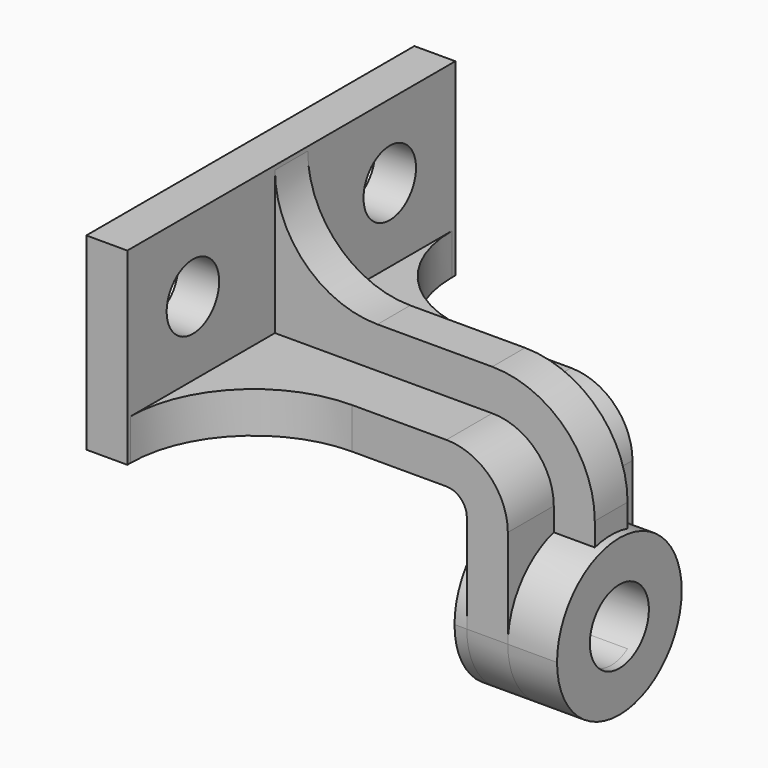
from build123d import *

# Parameters (mm, degrees)
F0_W      = 10
F0_H      = 36
F0_H_2    = 10
F0_W_2    = 58
F0_H_3    = 48
F1_DEPTH  = 50
F4_DEPTH  = 58.001
F2_R      = 8
F5_DEPTH  = 25
F6_R      = 15
F7_R      = 5
F9_DEPTH  = 5
F10_R     = 25
F13_DEPTH = 25
F12_R     = 9
F14_DEPTH = 25
F15_DEPTH = 25


# Not quite as in the source:
# - after a boolean that leaves OpenCascade's solid faulty, fix() repairs it


with BuildPart() as f1:
    # F0 (on Front) → F1 (new body, symmetric)
    with BuildSketch(Plane.XZ):
        with Locations((5, 28)):
            Rectangle(F0_W, F0_H)
        with Locations((5, 5)):
            Rectangle(F0_W, F0_H_2)
        with Locations((39, 5)):
            Rectangle(F0_W_2, F0_H_2)
        with Locations((73, 5)):
            Rectangle(F0_W, F0_H_2)
        with Locations((73, -24)):
            Rectangle(F0_W, F0_H_3)
    extrude(amount=F1_DEPTH, both=True)

    # F3 (on face) → F4 (cut, through all)
    with BuildSketch(Plane.XY.offset(10)):
        with BuildLine():
            Line((78, -19), (40, -19))
            ThreePointArc((40, -19), (18.7867965644, -27.7867965644), (10, -49))
            Line((10, -49), (10, -50))
            Line((10, -50), (78, -50))
            Line((78, -50), (78, -19))
        make_face()
        with BuildLine():
            ThreePointArc((10, 49), (18.7867965644, 27.7867965644), (40, 19))
            Line((40, 19), (78, 19))
            Line((78, 19), (78, 50))
            Line((78, 50), (10, 50))
            Line((10, 50), (10, 49))
        make_face()
    extrude(amount=-F4_DEPTH, mode=Mode.SUBTRACT)

    # F2 (on face) → F5 (cut)
    with BuildSketch(Plane.YZ.offset(10)):
        with Locations((30, 28)):
            Circle(F2_R)
        with Locations((-30, 28)):
            Circle(F2_R)
    extrude(amount=-F5_DEPTH, mode=Mode.SUBTRACT)

    # F6
    f6_edges = [f1.edges().sort_by_distance(p)[0] for p in [
        (78, 0, 10),
    ]]
    fillet(f6_edges, radius=F6_R)

    # F7
    f7_edges = [f1.edges().sort_by_distance(p)[0] for p in [
        (68, 0, 0),
    ]]
    fillet(f7_edges, radius=F7_R)

    # F8 (on Front) → F9 (join, symmetric)
    with BuildSketch(Plane.XZ):
        with BuildLine():
            ThreePointArc((35, 20), (17.3223304703, 27.3223304703), (10, 45))
            Line((10, 45), (10, 10))
            Line((10, 10), (40, 10))
            Line((40, 10), (63, 10))
            ThreePointArc((63, 10), (73.6066017178, 5.6066017178), (78, -5))
            Line((78, -5), (78, -48))
            Line((78, -48), (88, -48))
            Line((88, -48), (88, 20))
            Line((88, 20), (35, 20))
        make_face()
    extrude(amount=F9_DEPTH, both=True)

    # F10
    f10_edges = [f1.edges().sort_by_distance(p)[0] for p in [
        (88, 0, 20),
    ]]
    fillet(f10_edges, radius=F10_R)

    # F12 (on offset) → F13 (cut)
    with BuildSketch(Plane.YZ.offset(90)):
        with BuildLine():
            ThreePointArc((0, -48), (-13.4350288425, -42.4350288425), (-19, -29))
            Line((-19, -29), (-19, -48))
            Line((-19, -48), (-5, -48))
            Line((-5, -48), (0, -48))
        make_face()
        with BuildLine():
            Line((19, -48), (19, -29))
            ThreePointArc((19, -29), (13.4350288425, -42.4350288425), (0, -48))
            Line((0, -48), (5, -48))
            Line((5, -48), (19, -48))
        make_face()
    extrude(amount=-F13_DEPTH, mode=Mode.SUBTRACT)

    # F12 (on offset) → F14 (join)
    with BuildSketch(Plane.YZ.offset(90)):
        with BuildLine():
            ThreePointArc((0, -48), (13.4350288425, -42.4350288425), (19, -29))
            ThreePointArc((19, -29), (0, -10), (-19, -29))
            ThreePointArc((-19, -29), (-13.4350288425, -42.4350288425), (0, -48))
        make_face()
        with Locations((0, -29)):
            Circle(F12_R, mode=Mode.SUBTRACT)
    extrude(amount=-F14_DEPTH)

    add(f1.part.fix(), mode=Mode.REPLACE)

    # F12 (on offset) → F15 (cut)
    with BuildSketch(Plane.YZ.offset(90)):
        with Locations((0, -29)):
            Circle(F12_R)
    extrude(amount=-F15_DEPTH, mode=Mode.SUBTRACT)


solid = f1.part
